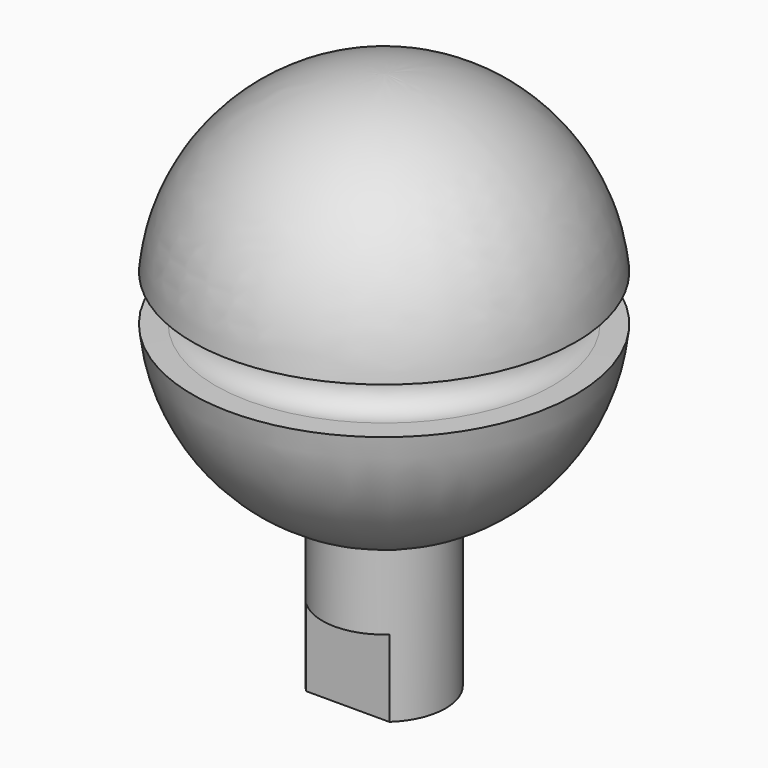
from build123d import *

# Parameters (mm, degrees)
F0_R      = 4
F1_DEPTH  = 10
F2_R      = 12.5
F3_DEPTH  = 25
F9_D      = 3.5
F9_DEPTH  = 13.5
F9_TIP    = 1.0515060833
F10_DEPTH = 5


# Not quite as in the source:
# - a fillet or chamfer that OpenCascade refuses, or shapes differently, is made with other operations: its cross-section is extruded or revolved along the edge and cut away or added


with BuildPart() as f1:
    # F0 (on Top) → F1 (new body)
    with BuildSketch(Plane.XY):
        Circle(F0_R)
    extrude(amount=F1_DEPTH)

    # F2 (on face) → F3 (join)
    with BuildSketch(Plane.XY.offset(10)):
        Circle(F2_R)
    extrude(amount=F3_DEPTH)

    # F4: fillet of radius 12.499 on 2 edges, made by hand

    # F4_s1 → F4_t2 (revolve, cut)
    with BuildSketch(Plane.XZ):
        with BuildLine():
            ThreePointArc((12.5, 22.501), (8.8391276581, 31.3391276581), (0.001, 35))
            Line((0.001, 35), (12.5, 35))
            Line((12.5, 35), (12.5, 22.501))
        make_face()
    revolve(axis=Axis((0, 0, 35), (0, 0, 1)), mode=Mode.SUBTRACT)

    # F4_s3 → F4_t4 (revolve, cut)
    with BuildSketch(Plane.XZ):
        with BuildLine():
            ThreePointArc((12.5, 21.84200152), (10.1550263443, 14.5536032049), (4, 10))
            Line((4, 10), (12.5, 10))
            Line((12.5, 10), (12.5, 21.84200152))
        make_face()
    revolve(axis=Axis((0, 0, 10), (0, 0, 1)), mode=Mode.SUBTRACT)

    # F5 (on Right) → F6 (revolve, cut)
    with BuildSketch(Plane.YZ):
        with BuildLine():
            Line((12.5007824972, 23.6938826144), (10.963675566, 23.7266744822))
            ThreePointArc((10.963675566, 23.7266744822), (9.463675566, 22.2266744822), (10.963675566, 20.7266744822))
            Line((10.963675566, 20.7266744822), (12.5007824972, 20.6938826144))
            Line((12.5007824972, 20.6938826144), (12.5007824972, 23.6938826144))
        make_face()
    revolve(axis=Axis((0, 0, 10), (0, 0, -1)), mode=Mode.SUBTRACT)

    # F9
    with Locations(Plane(origin=(0, 0, 0), x_dir=(1, 0, 0), z_dir=(0, 0, -1))):
        with Locations((0, 0)):
            Hole(F9_D / 2, depth=F9_DEPTH)
            with Locations((0, 0, -(F9_DEPTH + F9_TIP / 2))):  # 118° drill point
                Cone(0, F9_D / 2, F9_TIP, mode=Mode.SUBTRACT)

    # F7 (on face) → F10 (cut)
    with BuildSketch(Plane(origin=(0, 0, 0), x_dir=(1, 0, 0), z_dir=(0, 0, -1))):
        with BuildLine():
            ThreePointArc((-2.7013885318, -2.95), (0, -4), (2.7013885318, -2.95))
            Line((2.7013885318, -2.95), (-2.7013885318, -2.95))
        make_face()
        with BuildLine():
            Line((-2.7013885318, 2.95), (2.7013885318, 2.95))
            ThreePointArc((2.7013885318, 2.95), (0, 4), (-2.7013885318, 2.95))
        make_face()
    extrude(amount=-F10_DEPTH, mode=Mode.SUBTRACT)


solid = f1.part
